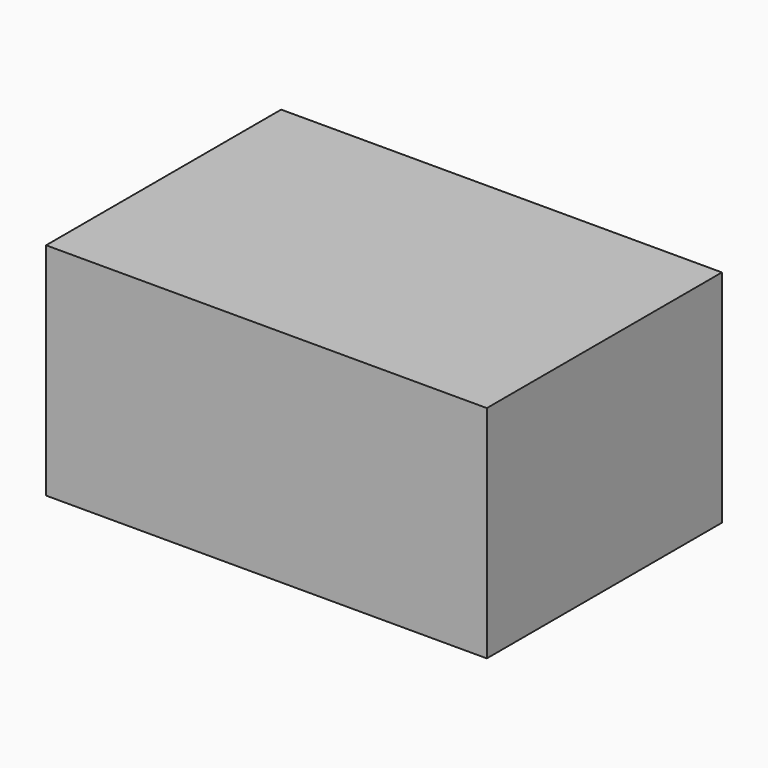
from build123d import *

# Parameters (mm, degrees)
F0_W     = 76.2
F0_H     = 50.8
F1_DEPTH = 38.1


# Not quite as in the source:
# - a feature of the source that left no trace in its solid (it failed there, or was rolled back) is left out


with BuildPart() as f1:
    # F0 (on Top) → F1 (new body)
    with BuildSketch(Plane.XY):
        Rectangle(F0_W, F0_H)
    extrude(amount=F1_DEPTH)


solid = f1.part
